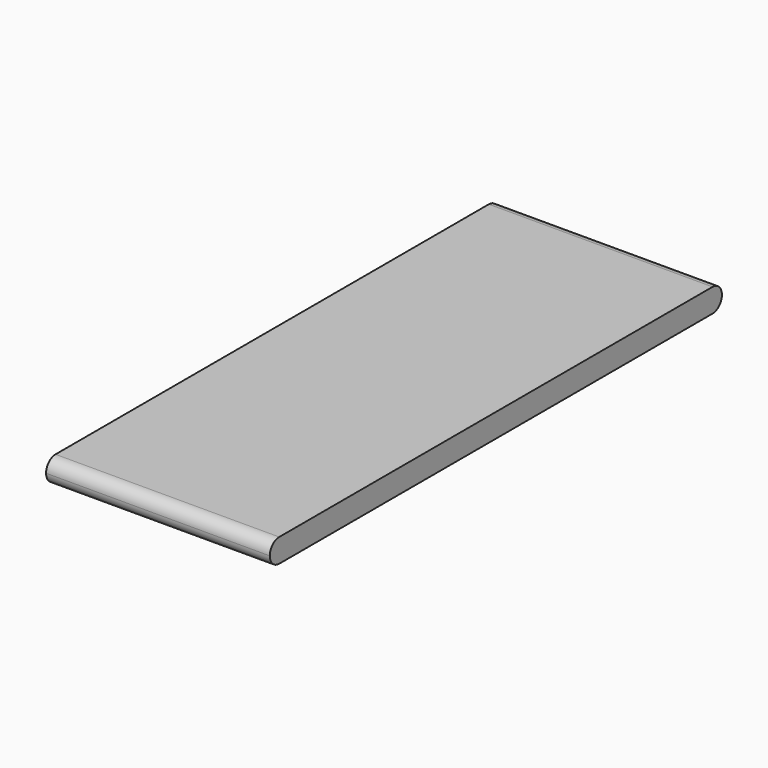
from build123d import *

# Parameters (mm, degrees)
F0_W     = 1219.2
F0_H     = 50.8
F1_DEPTH = 241.3
F2_R     = 25.39999


# Not quite as in the source:
# - a fillet or chamfer is up to 0.001 mm smaller than in the source, because OpenCascade refuses the exact size


with BuildPart() as f1:
    # F0 (on Right) → F1 (new body, symmetric)
    with BuildSketch(Plane.YZ):
        Rectangle(F0_W, F0_H)
    extrude(amount=F1_DEPTH, both=True)

    # F2 (radius 25.4 in the source; OpenCascade refuses exactly that, so slightly less here)
    f2_edges = [f1.edges().sort_by_distance(p)[0] for p in [
        (0, -609.6, 25.4),
        (0, -609.6, -25.4),
        (0, 609.6, -25.4),
        (0, 609.6, 25.4),
    ]]
    fillet(f2_edges, radius=F2_R)


solid = f1.part
